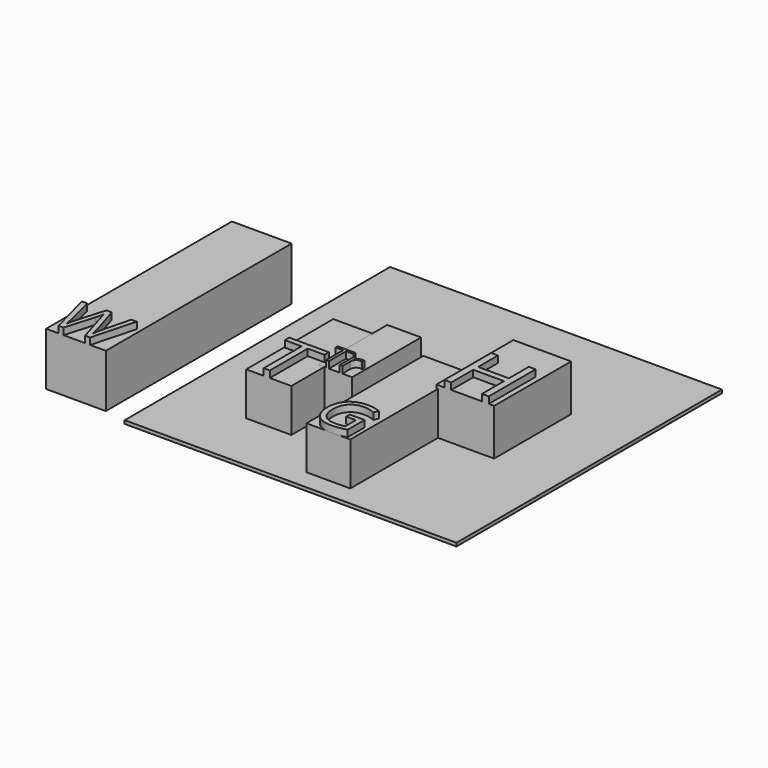
from build123d import *

# Parameters (mm, degrees)
F0_W          = 15240
F0_H          = 15240
F1_DEPTH      = 152.4
F2_W          = 2011.68
F2_H          = 6705.6
F3_DEPTH      = 2133.6
F4_TEXT_SIZE  = 2795.2132001737
F5_DEPTH      = 304.8
F6_W          = 2072.64
F6_H          = 4998.72
F7_DEPTH      = 2133.6
F8_TEXT_SIZE  = 3404.7474332649
F9_DEPTH      = 304.8
F10_W         = 1554.48
F10_H         = 3962.4
F11_DEPTH     = 2133.6
F12_TEXT_SIZE = 1535.7628897808
F13_DEPTH     = 304.8
F14_W         = 2651.76
F14_H         = 4419.6
F15_DEPTH     = 2133.6
F16_TEXT_SIZE = 3761.3617021277
F17_DEPTH     = 304.8
F18_W         = 2743.2
F18_H         = 10668
F19_DEPTH     = 2438.4
F20_TEXT_SIZE = 2807.6891092276
F21_DEPTH     = 304.8


# Not quite as in the source:
# - Text() gives the source's letters only with a copy of the font that has no kerning and outlines rounded to 1/6400 em; it was checked with that copy


with BuildPart() as f1:
    # F0 (on Top) → F1 (new body)
    with BuildSketch(Plane.XY):
        Rectangle(F0_W, F0_H)
    extrude(amount=F1_DEPTH)


with BuildPart() as f3:
    # F2 (on Top) → F3 (new body)
    with BuildSketch(Plane.XY):
        with Locations((1005.84, -3352.8)):
            Rectangle(F2_W, F2_H)
    extrude(amount=F3_DEPTH)

    # F4 (on face) → F5 (join)
    with BuildSketch(Plane.XY.offset(2133.6)):
        with Locations((0, -6705.6)):
            Text('G', F4_TEXT_SIZE, font='Open Sans', text_align=(TextAlign.LEFT, TextAlign.BOTTOM))
    extrude(amount=F5_DEPTH)


with BuildPart() as f7:
    # F6 (on face) → F7 (new body)
    with BuildSketch(Plane.XY):
        with Locations((-3269.4586122044, -2284.5779767549)):
            Rectangle(F6_W, F6_H)
    extrude(amount=F7_DEPTH)

    # F8 (on face) → F9 (join)
    with BuildSketch(Plane.XY.offset(2133.6)):
        with Locations((-4305.7786122044, -4783.9379767549)):
            Text('T', F8_TEXT_SIZE, font='Open Sans', text_align=(TextAlign.LEFT, TextAlign.BOTTOM))
    extrude(amount=F9_DEPTH)


with BuildPart() as f11:
    # F10 (on Top) → F11 (new body)
    with BuildSketch(Plane.XY):
        with Locations((-1733.5387922356, -910.4380169949)):
            Rectangle(F10_W, F10_H)
    extrude(amount=F11_DEPTH)

    # F12 (on face) → F13 (join)
    with BuildSketch(Plane.XY.offset(2133.6)):
        with Locations((-2510.7787922356, -2891.6380169949)):
            Text('Tr', F12_TEXT_SIZE, font='Open Sans', text_align=(TextAlign.LEFT, TextAlign.BOTTOM))
    extrude(amount=F13_DEPTH)


with BuildPart() as f15:
    # F14 (on face) → F15 (new body)
    with BuildSketch(Plane.XY.offset(152.4)):
        with Locations((3265.6750679016, 537.5610150141)):
            Rectangle(F14_W, F14_H)
    extrude(amount=F15_DEPTH)

    # F16 (on face) → F17 (join)
    with BuildSketch(Plane.XY.offset(2286)):
        with Locations((1939.7950679016, -1672.2389849859)):
            Text('H', F16_TEXT_SIZE, font='Open Sans', text_align=(TextAlign.LEFT, TextAlign.BOTTOM))
    extrude(amount=F17_DEPTH)


with BuildPart() as f19:
    # F18 (on face) → F19 (new body)
    with BuildSketch(Plane.XY.offset(152.4)):
        with Locations((-9960.9456062317, -2157.4690115684)):
            Rectangle(F18_W, F18_H)
    extrude(amount=F19_DEPTH)

    # F20 (on face) → F21 (join)
    with BuildSketch(Plane.XY.offset(2590.8)):
        with Locations((-11332.5456062317, -7491.4690115684)):
            Text('W', F20_TEXT_SIZE, font='Open Sans', text_align=(TextAlign.LEFT, TextAlign.BOTTOM))
    extrude(amount=F21_DEPTH)


solid = Compound([f1.part, f3.part, f7.part, f11.part, f15.part, f19.part])
